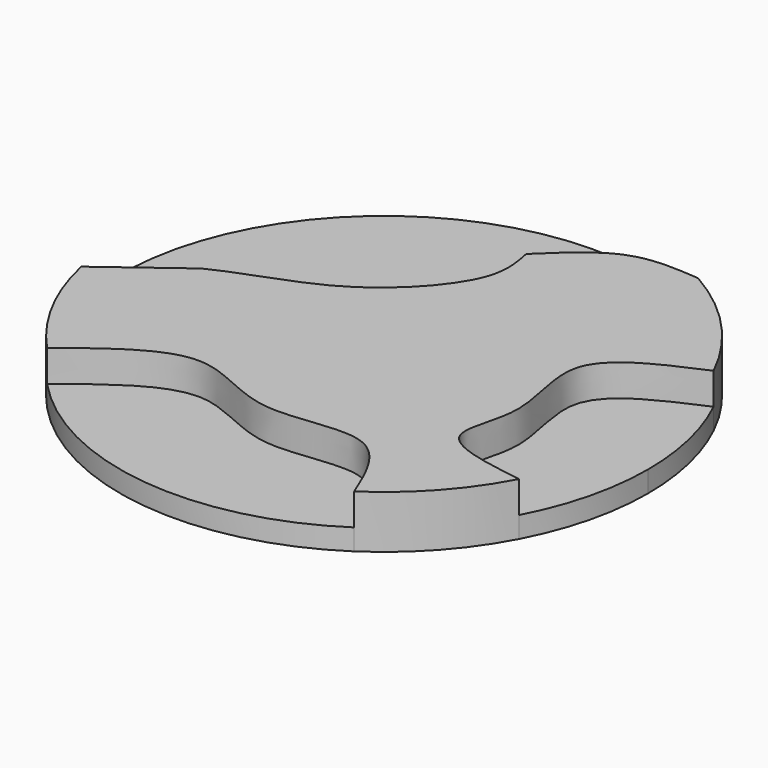
from build123d import *

# Parameters (mm, degrees)
F1_DEPTH = 2
F2_DEPTH = 5


with BuildPart() as f1:
    # F0 (on Top) → F1 (new body)
    with BuildSketch(Plane.XY):
        with BuildLine():
            ThreePointArc((22.1188925873, -11.6513772023), (24.2690370089, -6.001153444), (25, 0))
            ThreePointArc((25, 0), (24.3701069704, 5.5765478793), (22.5121691, 10.8720854676))
            add(Edge.make_bspline(
                [(22.5121691, 10.8720854676), (18.8895611428, 9.3055197167), (11.9102659407, 6.2896821538), (16.4364178682, -3.0658471403), (12.2521680449, -10.2063529762), (18.6615851191, -11.1474987265), (22.1188925873, -11.6513772023)],
                knots=[0, 0, 0, 0, 0.2780136343, 0.5343531988, 0.7479805585, 1, 1, 1, 1], degree=3))
        make_face()
    extrude(amount=F1_DEPTH)


with BuildPart() as f1b:
    # F0 (on Top) → F1, piece 2 (new body)
    with BuildSketch(Plane.XY):
        with BuildLine():
            add(Edge.make_bspline(
                [(0, 16.8172493577), (1.9144161531, 18.6824676113), (5.5934798745, 22.2645311542), (10.1584208321, 21.9120162799), (12.34633467, 21.7386296766)],
                knots=[0, 0, 0, 0, 0.5203475383, 1, 1, 1, 1], degree=3))
            ThreePointArc((12.34633467, 21.7386296766), (-14.8165901958, 20.1362522573), (-24.4273769181, -5.3200805351))
            add(Edge.make_bspline(
                [(-24.4273769181, -5.3200805351), (-22.2453911763, -3.3574319676), (-20.0634054345, -1.3947834001), (-17.3023622483, 0)],
                knots=[0, 0, 0, 0, 0.254891956, 0.254891956, 0.254891956, 0.254891956], degree=3))
            add(Edge.make_bspline(
                [(-17.3023622483, 0), (-14.1903788127, 1.5720662607), (-6.6472654424, 3.2397841474), (-0.8648455283, 9.7284013886), (0, 12.2895278037)],
                knots=[0.254891956, 0.254891956, 0.254891956, 0.254891956, 0.542181756, 0.8181160828, 0.8181160828, 0.8181160828, 0.8181160828], degree=3))
            Line((0, 12.2895278037), (0, 16.8172493577))
        make_face()
        with BuildLine():
            add(Edge.make_bspline(
                [(-24.4273769181, -5.3200805351), (-22.2453911763, -3.3574319676), (-20.0634054345, -1.3947834001), (-17.3023622483, 0)],
                knots=[0, 0, 0, 0, 0.254891956, 0.254891956, 0.254891956, 0.254891956], degree=3))
            Line((-24.4273769181, -5.3200805351), (-17.3023622483, 0))
        make_face()
    extrude(amount=F1_DEPTH)


with BuildPart() as f1c:
    # F0 (on Top) → F1, piece 3 (new body)
    with BuildSketch(Plane.XY):
        with BuildLine():
            ThreePointArc((-18.2737018092, -17.0608271249), (-2.9135456355, -24.8296446175), (13.8278126154, -20.8276642539))
            add(Edge.make_bspline(
                [(-18.2737018092, -17.0608271249), (-14.8332101277, -14.3400323801), (-8.3808524987, -9.228978734), (-0.4412585546, -15.998889193), (10.2263751779, -12.0238586347), (12.6576888155, -17.9664290501), (13.8278126154, -20.8276642539)],
                knots=[0, 0, 0, 0, 0.2769679297, 0.5181649262, 0.767240907, 1, 1, 1, 1], degree=3))
        make_face()
    extrude(amount=F1_DEPTH)


with BuildPart() as f2:
    # F0 (on Top) → F2 (new body)
    with BuildSketch(Plane.XY):
        with BuildLine():
            add(Edge.make_bspline(
                [(22.5121691, 10.8720854676), (18.8895611428, 9.3055197167), (11.9102659407, 6.2896821538), (16.4364178682, -3.0658471403), (12.2521680449, -10.2063529762), (18.6615851191, -11.1474987265), (22.1188925873, -11.6513772023)],
                knots=[0, 0, 0, 0, 0.2780136343, 0.5343531988, 0.7479805585, 1, 1, 1, 1], degree=3))
            ThreePointArc((22.5121691, 10.8720854676), (18.2564856156, 17.0792486067), (12.34633467, 21.7386296766))
            add(Edge.make_bspline(
                [(0, 16.8172493577), (1.9144161531, 18.6824676113), (5.5934798745, 22.2645311542), (10.1584208321, 21.9120162799), (12.34633467, 21.7386296766)],
                knots=[0, 0, 0, 0, 0.5203475383, 1, 1, 1, 1], degree=3))
            add(Edge.make_bspline(
                [(0, 12.2895278037), (0.5700685894, 13.9777110398), (0.2850342947, 15.3974801988), (0, 16.8172493577)],
                knots=[0.8181160828, 0.8181160828, 0.8181160828, 0.8181160828, 1, 1, 1, 1], degree=3))
            add(Edge.make_bspline(
                [(-17.3023622483, 0), (-14.1903788127, 1.5720662607), (-6.6472654424, 3.2397841474), (-0.8648455283, 9.7284013886), (0, 12.2895278037)],
                knots=[0.254891956, 0.254891956, 0.254891956, 0.254891956, 0.542181756, 0.8181160828, 0.8181160828, 0.8181160828, 0.8181160828], degree=3))
            Line((-17.3023622483, 0), (-24.4273769181, -5.3200805351))
            ThreePointArc((-24.4273769181, -5.3200805351), (-22.1428727527, -11.6057393672), (-18.2737018092, -17.0608271249))
            add(Edge.make_bspline(
                [(-18.2737018092, -17.0608271249), (-14.8332101277, -14.3400323801), (-8.3808524987, -9.228978734), (-0.4412585546, -15.998889193), (10.2263751779, -12.0238586347), (12.6576888155, -17.9664290501), (13.8278126154, -20.8276642539)],
                knots=[0, 0, 0, 0, 0.2769679297, 0.5181649262, 0.767240907, 1, 1, 1, 1], degree=3))
            ThreePointArc((13.8278126154, -20.8276642539), (18.549729506, -16.7602963951), (22.1188925873, -11.6513772023))
        make_face()
    extrude(amount=F2_DEPTH)


solid = Compound([f1.part, f1b.part, f1c.part, f2.part])
